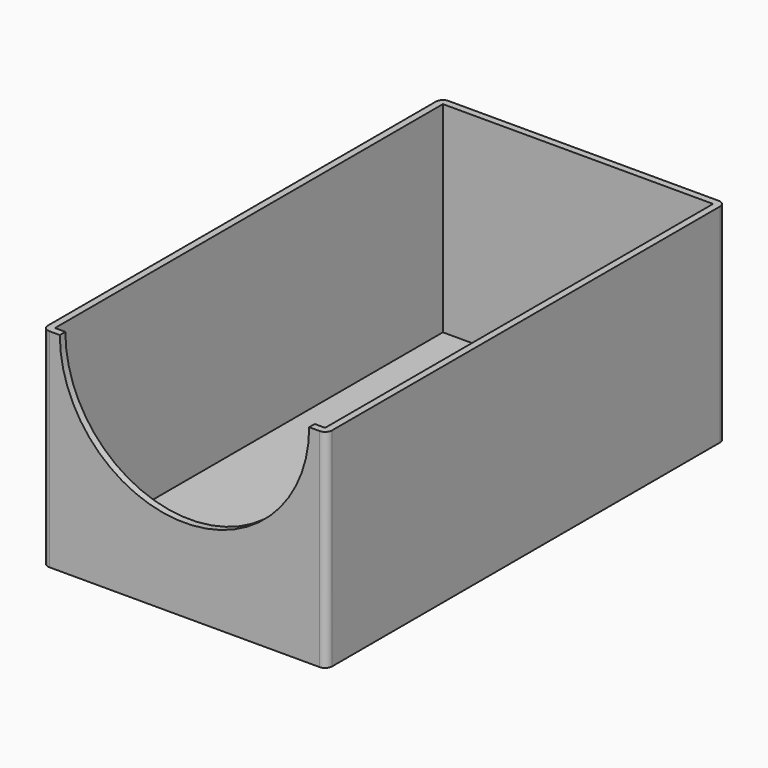
from build123d import *

# Parameters (mm, degrees)
F0_W     = 78
F0_H     = 140
F1_DEPTH = 2
F0_W_2   = 82
F0_H_2   = 144
F2_DEPTH = 60
F4_DEPTH = 25
F5_R     = 2


# Not quite as in the source:
# - a feature names something its author has since deleted; it is built from what else it names


with BuildPart() as f1:
    # F0 (on Top) → F1 (new body)
    with BuildSketch(Plane.XY):
        Rectangle(F0_W, F0_H)
    extrude(amount=F1_DEPTH)

    # F0 (on Top) → F2 (join)
    with BuildSketch(Plane.XY):
        Rectangle(F0_W_2, F0_H_2)
        Rectangle(F0_W, F0_H, mode=Mode.SUBTRACT)
    extrude(amount=F2_DEPTH)

    # F3 (on face) → F4 (cut)
    with BuildSketch(Plane(origin=(0, -70, 0), x_dir=(-1, 0, 0), z_dir=(0, 1, 0))):
        with BuildLine():
            Line((36, 60), (-36, 60))
            ThreePointArc((-36, 60), (0, 24), (36, 60))
        make_face()
    extrude(amount=-F4_DEPTH, mode=Mode.SUBTRACT)

    # F5
    f5_edges = [f1.edges().sort_by_distance(p)[0] for p in [
        (-41, 72, 30),
        (41, 72, 30),
        (-41, -72, 30),
        (41, -72, 30),
    ]]
    fillet(f5_edges, radius=F5_R)


solid = f1.part
